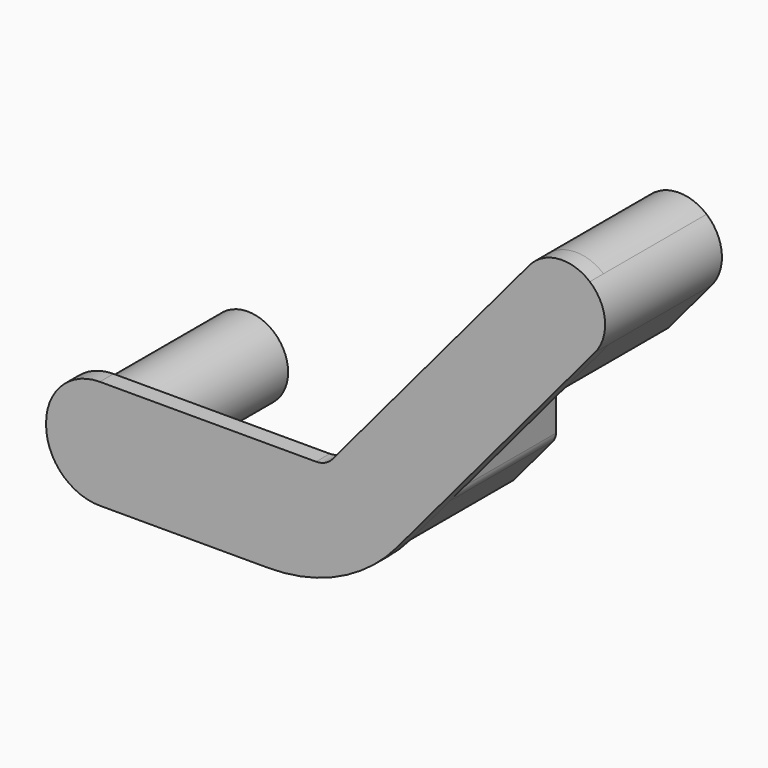
from build123d import *

# Parameters (mm, degrees)
F1_DEPTH    = 4
F2_R        = 9.99999
F3_R        = 12.5
F6_DEPTH    = 30
F4_R        = 9.3845657054
F7_DEPTH    = 43.1
F8_T1_DEPTH = 50.6060806459
F8_T3_DEPTH = 32.729776757
F8_T5_DEPTH = 33.6001001543
F9_R        = 39
F10_R       = 5


# Not quite as in the source:
# - a fillet or chamfer that OpenCascade refuses, or shapes differently, is made with other operations: its cross-section is extruded or revolved along the edge and cut away or added
# - a fillet or chamfer is up to 0.001 mm smaller than in the source, because OpenCascade refuses the exact size
# - ends of sketch curves that miss each other by under 0.0002 mm in the source are joined


with BuildPart() as f1:
    # F0 (on Front) → F1 (new body)
    with BuildSketch(Plane.XZ):
        Polygon((-70, 0), (0, 0), (64.2787609687, 76.6044443119), (48.9578721063, 89.4601965056), (-4.7950151547, 25.4), (-70, 25.4), align=None)
    extrude(amount=F1_DEPTH)

    # F2 (radius 10 in the source; OpenCascade refuses exactly that, so slightly less here)
    f2_edges = [f1.edges().sort_by_distance(p)[0] for p in [
        (64.278761, -2, 76.604444),
        (48.957872, -2, 89.460197),
    ]]
    fillet(f2_edges, radius=F2_R)

    # F3
    f3_edges = [f1.edges().sort_by_distance(p)[0] for p in [
        (-70, -2, 0),
        (-70, -2, 25.4),
    ]]
    fillet(f3_edges, radius=F3_R)

    # F5 (on face) → F6 (join)
    with BuildSketch(Plane(origin=(0, 0, 0), x_dir=(-1, 0, 0), z_dir=(0, 1, 0))):
        with BuildLine():
            Line((-42.5299960094, 50.6852755372), (-42.5299960094, 81.7997520744))
            ThreePointArc((-42.5299960094, 81.7997520744), (-49.3188826521, 85.3338270849), (-56.618308877, 83.0323268366))
            ThreePointArc((-56.618308877, 83.0323268366), (-60.1523915479, 76.2434337661), (-57.8508912997, 68.9440075412))
            Line((-57.8508912997, 68.9440075412), (-42.5299960094, 50.6852755372))
        make_face()
        Polygon((-6.5299960094, 38.896622741), (-21.5299960094, 56.77292663), (-21.5299960094, 25.6584500928), (-6.5299960094, 7.7821462038), align=None)
    extrude(amount=F6_DEPTH)

    # F4 (on face) → F7 (join)
    with BuildSketch(Plane.XZ.offset(4)):
        with Locations((-57.5, 12.9)):
            Circle(F4_R)
    extrude(amount=-F7_DEPTH)

    # F8: fillet of radius 3 on 6 edges, made by hand

    # F8_s2 → F8_t1 (cut)
    with BuildSketch(Plane.XZ.offset(-50.6060806459)):
        with BuildLine():
            ThreePointArc((16.2318626801, 50.4588572007), (19.5560564394, 51.349572234), (21.5299960094, 48.5304943716))
            Line((21.5299960094, 48.5304943716), (21.5299960094, 56.77292663))
            Line((21.5299960094, 56.77292663), (16.2318626801, 50.4588572007))
        make_face()
        with BuildLine():
            ThreePointArc((11.8281293388, 14.0962156331), (8.5039355794, 13.2055005998), (6.5299960094, 16.0245784622))
            Line((6.5299960094, 16.0245784622), (6.5299960094, 7.7821462038))
            Line((6.5299960094, 7.7821462038), (11.8281293388, 14.0962156331))
        make_face()
        with BuildLine():
            ThreePointArc((47.8281293388, 56.9993449665), (44.5039355794, 56.1086299332), (42.5299960094, 58.9277077956))
            Line((42.5299960094, 58.9277077956), (42.5299960094, 50.6852755372))
            Line((42.5299960094, 50.6852755372), (47.8281293388, 56.9993449665))
        make_face()
    extrude(amount=F8_T1_DEPTH, mode=Mode.SUBTRACT)

    # F8_s4 → F8_t3 (cut)
    with BuildSketch(Plane.XZ.offset(-32.729776757)):
        with BuildLine():
            ThreePointArc((20.8281293388, 24.8219979665), (21.3490738718, 25.7243003656), (21.5299960094, 26.7503607956))
            Line((21.5299960094, 26.7503607956), (21.5299960094, 25.6584500928))
            Line((21.5299960094, 25.6584500928), (20.8281293388, 24.8219979665))
        make_face()
        with BuildLine():
            ThreePointArc((6.5299960094, 37.8047120382), (6.7109181471, 38.8307724682), (7.2318626801, 39.7330748673))
            Line((7.2318626801, 39.7330748673), (6.5299960094, 38.896622741))
            Line((6.5299960094, 38.896622741), (6.5299960094, 37.8047120382))
        make_face()
    extrude(amount=F8_T3_DEPTH, mode=Mode.SUBTRACT)

    # F8_s6 → F8_t5 (cut)
    with BuildSketch(Plane.XZ.offset(-33.6001001543)):
        with BuildLine():
            ThreePointArc((42.5299960094, 80.5949283764), (42.7921129807, 81.8213037352), (43.5326603567, 82.8333765643))
            ThreePointArc((43.5326603567, 82.8333765643), (43.0126982288, 82.3346362508), (42.5299960094, 81.7997520744))
            Line((42.5299960094, 81.7997520744), (42.5299960094, 80.5949283764))
        make_face()
    extrude(amount=F8_T5_DEPTH, mode=Mode.SUBTRACT)

    # F9
    f9_edges = [f1.edges().sort_by_distance(p)[0] for p in [
        (0, -2, 0),
    ]]
    fillet(f9_edges, radius=F9_R)

    # F10
    f10_edges = [f1.edges().sort_by_distance(p)[0] for p in [
        (-4.795015, -2, 25.4),
    ]]
    fillet(f10_edges, radius=F10_R)


solid = f1.part
